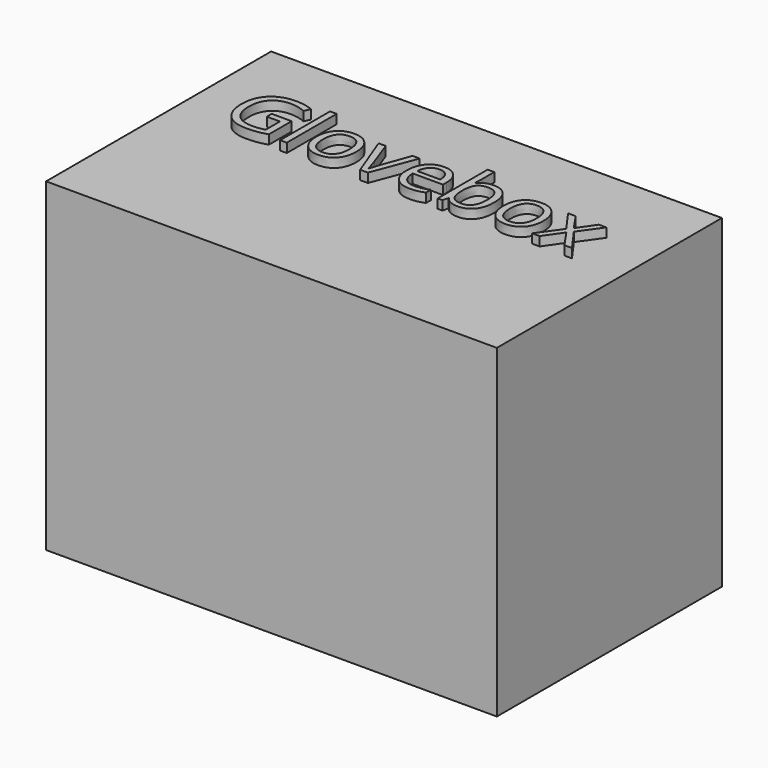
from build123d import *

# Parameters (mm, degrees)
F0_W         = 1250
F0_H         = 780
F1_DEPTH     = 900
F2_TEXT_SIZE = 227.6889565918
F3_DEPTH     = 25.4


# Not quite as in the source:
# - Text() gives the source's letters only with a copy of the font that has no kerning and outlines rounded to 1/6400 em; it was checked with that copy


with BuildPart() as f1:
    # F0 (on Top) → F1 (new body)
    with BuildSketch(Plane.XY):
        Rectangle(F0_W, F0_H)
    extrude(amount=F1_DEPTH)

    # F2 (on face) → F3 (join)
    with BuildSketch(Plane.XY.offset(900)):
        with Locations((-504.6334382464, 39.1133725643)):
            Text('Glovebox', F2_TEXT_SIZE, font='Open Sans', text_align=(TextAlign.LEFT, TextAlign.BOTTOM))
    extrude(amount=F3_DEPTH)


solid = f1.part
